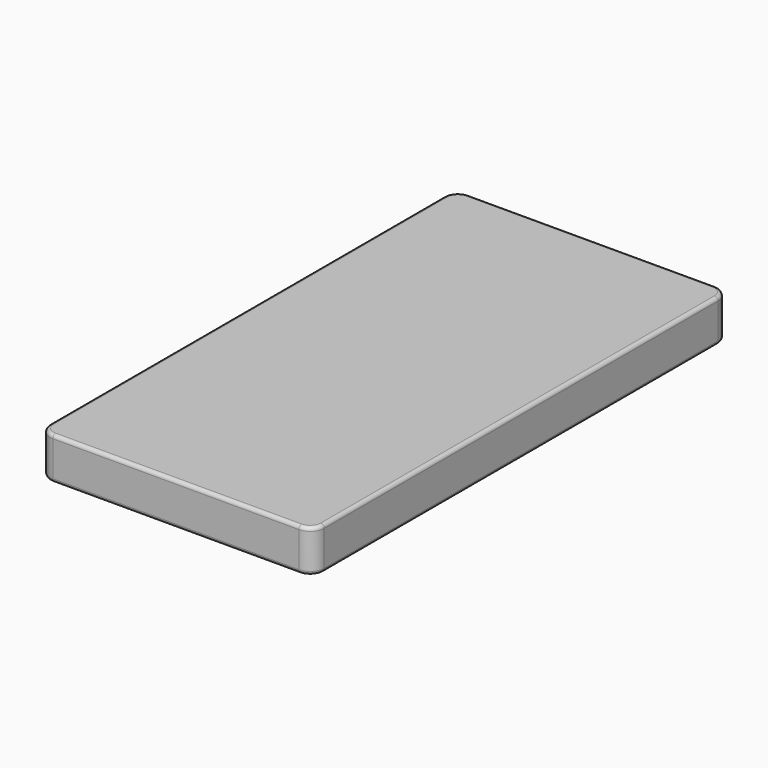
from build123d import *

# Parameters (mm, degrees)
F0_W         = 990.6
F0_H         = 1879.6
F1_DEPTH     = 152.4
F2_R         = 12.7
F3_T1_DEPTH  = 152.4
F3_T4_ANGLE  = 90
F3_T6_ANGLE  = 90
F3_T8_ANGLE  = 90
F3_T10_ANGLE = 90
F3_T12_ANGLE = 90
F3_T14_ANGLE = 90
F3_T16_ANGLE = 90
F3_T18_ANGLE = 90


# Not quite as in the source:
# - a fillet or chamfer that OpenCascade refuses, or shapes differently, is made with other operations: its cross-section is extruded or revolved along the edge and cut away or added


with BuildPart() as f1:
    # F0 (on Top) → F1 (new body)
    with BuildSketch(Plane.XY):
        Rectangle(F0_W, F0_H)
    extrude(amount=F1_DEPTH)

    # F2
    f2_edges = [f1.edges().sort_by_distance(p)[0] for p in [
        (-495.3, 0, 152.4),
        (0, -939.8, 152.4),
        (495.3, 0, 152.4),
        (0, 939.8, 152.4),
        (495.3, 0, 0),
        (0, -939.8, 0),
        (-495.3, 0, 0),
        (0, 939.8, 0),
    ]]
    fillet(f2_edges, radius=F2_R)

    # F3: fillet of radius 50.8 on 4 edges, made by hand

    # F3_s2 → F3_t1 (cut)
    with BuildSketch(Plane.XY):
        with BuildLine():
            ThreePointArc((-495.3, -889), (-480.4210244843, -924.9210244843), (-444.5, -939.8))
            Line((-444.5, -939.8), (-444.5, -940.816))
            Line((-444.5, -940.816), (-496.316, -940.816))
            Line((-496.316, -940.816), (-496.316, -889))
            Line((-496.316, -889), (-495.3, -889))
        make_face()
        with BuildLine():
            ThreePointArc((495.3, -889), (480.4210244843, -924.9210244843), (444.5, -939.8))
            Line((444.5, -939.8), (444.5, -940.816))
            Line((444.5, -940.816), (496.316, -940.816))
            Line((496.316, -940.816), (496.316, -889))
            Line((496.316, -889), (495.3, -889))
        make_face()
        with BuildLine():
            ThreePointArc((444.5, 939.8), (480.4210244843, 924.9210244843), (495.3, 889))
            Line((495.3, 889), (496.316, 889))
            Line((496.316, 889), (496.316, 940.816))
            Line((496.316, 940.816), (444.5, 940.816))
            Line((444.5, 940.816), (444.5, 939.8))
        make_face()
        with BuildLine():
            ThreePointArc((-444.5, 939.8), (-480.4210244843, 924.9210244843), (-495.3, 889))
            Line((-495.3, 889), (-496.316, 889))
            Line((-496.316, 889), (-496.316, 940.816))
            Line((-496.316, 940.816), (-444.5, 940.816))
            Line((-444.5, 940.816), (-444.5, 939.8))
        make_face()
    extrude(amount=F3_T1_DEPTH, mode=Mode.SUBTRACT)

    # F3_s3 → F3_t4 (revolve, cut)
    with BuildSketch(Plane.XZ.offset(-889)):
        with BuildLine():
            ThreePointArc((-482.6, 0), (-491.5802561211, 3.7197438789), (-495.3, 12.7))
            Line((-495.3, 12.7), (-495.3, 0))
            Line((-495.3, 0), (-482.6, 0))
        make_face()
    revolve(axis=Axis((-444.5, 889, 0), (0, 0, -1)), revolution_arc=F3_T4_ANGLE, mode=Mode.SUBTRACT)

    # F3_s5 → F3_t6 (revolve, cut)
    with BuildSketch(Plane.YZ.offset(-444.5)):
        with BuildLine():
            ThreePointArc((927.1, 152.4), (936.0802561211, 148.6802561211), (939.8, 139.7))
            Line((939.8, 139.7), (939.8, 152.4))
            Line((939.8, 152.4), (927.1, 152.4))
        make_face()
    revolve(axis=Axis((-444.5, 889, 152.4), (0, 0, 1)), revolution_arc=F3_T6_ANGLE, mode=Mode.SUBTRACT)

    # F3_s7 → F3_t8 (revolve, cut)
    with BuildSketch(Plane.YZ.offset(444.5)):
        with BuildLine():
            ThreePointArc((927.1, 0), (936.0802561211, 3.7197438789), (939.8, 12.7))
            Line((939.8, 12.7), (939.8, 0))
            Line((939.8, 0), (927.1, 0))
        make_face()
    revolve(axis=Axis((444.5, 889, 0), (0, 0, -1)), revolution_arc=F3_T8_ANGLE, mode=Mode.SUBTRACT)

    # F3_s9 → F3_t10 (revolve, cut)
    with BuildSketch(Plane.XZ.offset(-889)):
        with BuildLine():
            ThreePointArc((482.6, 152.4), (491.5802561211, 148.6802561211), (495.3, 139.7))
            Line((495.3, 139.7), (495.3, 152.4))
            Line((495.3, 152.4), (482.6, 152.4))
        make_face()
    revolve(axis=Axis((444.5, 889, 152.4), (0, 0, 1)), revolution_arc=F3_T10_ANGLE, mode=Mode.SUBTRACT)

    # F3_s11 → F3_t12 (revolve, cut)
    with BuildSketch(Plane.XZ.offset(889)):
        with BuildLine():
            ThreePointArc((482.6, 0), (491.5802561211, 3.7197438789), (495.3, 12.7))
            Line((495.3, 12.7), (495.3, 0))
            Line((495.3, 0), (482.6, 0))
        make_face()
    revolve(axis=Axis((444.5, -889, 0), (0, 0, -1)), revolution_arc=F3_T12_ANGLE, mode=Mode.SUBTRACT)

    # F3_s13 → F3_t14 (revolve, cut)
    with BuildSketch(Plane.YZ.offset(444.5)):
        with BuildLine():
            ThreePointArc((-927.1, 152.4), (-936.0802561211, 148.6802561211), (-939.8, 139.7))
            Line((-939.8, 139.7), (-939.8, 152.4))
            Line((-939.8, 152.4), (-927.1, 152.4))
        make_face()
    revolve(axis=Axis((444.5, -889, 152.4), (0, 0, 1)), revolution_arc=F3_T14_ANGLE, mode=Mode.SUBTRACT)

    # F3_s15 → F3_t16 (revolve, cut)
    with BuildSketch(Plane.YZ.offset(-444.5)):
        with BuildLine():
            ThreePointArc((-927.1, 0), (-936.0802561211, 3.7197438789), (-939.8, 12.7))
            Line((-939.8, 12.7), (-939.8, 0))
            Line((-939.8, 0), (-927.1, 0))
        make_face()
    revolve(axis=Axis((-444.5, -889, 0), (0, 0, -1)), revolution_arc=F3_T16_ANGLE, mode=Mode.SUBTRACT)

    # F3_s17 → F3_t18 (revolve, cut)
    with BuildSketch(Plane.XZ.offset(889)):
        with BuildLine():
            ThreePointArc((-482.6, 152.4), (-491.5802561211, 148.6802561211), (-495.3, 139.7))
            Line((-495.3, 139.7), (-495.3, 152.4))
            Line((-495.3, 152.4), (-482.6, 152.4))
        make_face()
    revolve(axis=Axis((-444.5, -889, 152.4), (0, 0, 1)), revolution_arc=F3_T18_ANGLE, mode=Mode.SUBTRACT)


solid = f1.part
